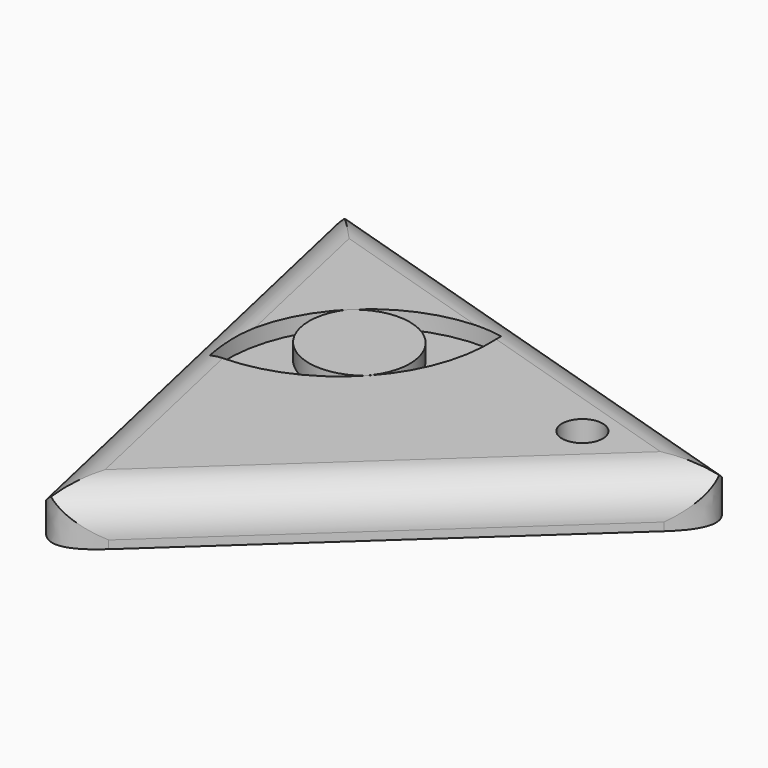
from build123d import *

# Parameters (mm, degrees)
F1_DEPTH    = 6
F3_DEPTH    = 2
F5_DEPTH    = 2
F6_T1_DEPTH = 95.6484477973
F6_T3_DEPTH = 95.6484477973
F6_T5_DEPTH = 95.6484477973
F7_T1_DEPTH = 44.3012701892
F8_R        = 2.5
F9_DEPTH    = 32.8


# Not quite as in the source:
# - a fillet or chamfer that OpenCascade refuses, or shapes differently, is made with other operations: its cross-section is extruded or revolved along the edge and cut away or added
# - a feature of the source that left no trace in its solid (it failed there, or was rolled back) is left out


with BuildPart() as f1:
    # F0 (on Top) → F1 (new body)
    with BuildSketch(Plane.XY):
        Polygon((-12.152816169, -38.9364026487), (39.7963219102, 8.9435537945), (-27.6435057413, 29.9928488542), align=None)
    extrude(amount=F1_DEPTH)

    # F2 (on face) → F3 (cut)
    with BuildSketch(Plane.XY.offset(6)):
        with BuildLine():
            ThreePointArc((-16.4638161659, -4.259868525), (-1.9528341067, 1.3079860402), (3.1085531227, 16.0032901913))
            ThreePointArc((3.1085531227, 16.0032901913), (-11.8846429173, 10.9012104958), (-16.4638161659, -4.259868525))
        make_face()
    extrude(amount=-F3_DEPTH, mode=Mode.SUBTRACT)

    # F6: fillet of radius 5 on 3 edges, made by hand

    # F6_s2 → F6_t1 (cut)
    with BuildSketch(Plane(origin=(-10.4861497959, 46.660444211, 0), x_dir=(0, 0, 1), z_dir=(0.2192644008, -0.9756654768, 0))):
        with BuildLine():
            ThreePointArc((1, 20.3944501768), (4.5355339059, 18.9299840827), (6, 15.3944501768))
            Line((6, 15.3944501768), (6, 20.3944501768))
            Line((6, 20.3944501768), (1, 20.3944501768))
        make_face()
    extrude(amount=F6_T1_DEPTH, mode=Mode.SUBTRACT)

    # F6_s4 → F6_t3 (cut)
    with BuildSketch(Plane(origin=(45.6522049365, -14.2489499944, 0), x_dir=(0, 0, 1), z_dir=(-0.9545832889, 0.2979441972, 0))):
        with BuildLine():
            ThreePointArc((1, 20.3944501768), (4.5355339059, 18.9299840827), (6, 15.3944501768))
            Line((6, 15.3944501768), (6, 20.3944501768))
            Line((6, 20.3944501768), (1, 20.3944501768))
        make_face()
    extrude(amount=F6_T3_DEPTH, mode=Mode.SUBTRACT)

    # F6_s6 → F6_t5 (cut)
    with BuildSketch(Plane(origin=(-35.1660551406, -32.4114942166, 0), x_dir=(0, 0, 1), z_dir=(0.7353188881, 0.6777212796, 0))):
        with BuildLine():
            ThreePointArc((1, 20.3944501768), (4.5355339059, 18.9299840827), (6, 15.3944501768))
            Line((6, 15.3944501768), (6, 20.3944501768))
            Line((6, 20.3944501768), (1, 20.3944501768))
        make_face()
    extrude(amount=F6_T5_DEPTH, mode=Mode.SUBTRACT)

    # F7: fillet of radius 5 on 3 edges, made by hand

    # F7_s2 → F7_t1 (cut)
    with BuildSketch(Plane.XY.offset(-21.6506350946)):
        with BuildLine():
            add(Edge.make_bspline(
                [(-25.7446203291, 21.5433379695), (-27.6435057413, 29.9928488542), (-19.3765719594, 27.4125764177)],
                knots=[0, 0, 0, 1, 1, 1], degree=2, weights=[1, 1, 1]))
            Line((-19.3765719594, 27.4125764177), (-27.6435057413, 29.9928488542))
            Line((-27.6435057413, 29.9928488542), (-25.7446203291, 21.5433379695))
        make_face()
        with BuildLine():
            add(Edge.make_bspline(
                [(-14.0517015812, -30.4868917639), (-12.152816169, -38.9364026487), (-5.7847677993, -33.0671642005)],
                knots=[0, 0, 0, 1, 1, 1], degree=2, weights=[1, 1, 1]))
            Line((-5.7847677993, -33.0671642005), (-12.152816169, -38.9364026487))
            Line((-12.152816169, -38.9364026487), (-14.0517015812, -30.4868917639))
        make_face()
        with BuildLine():
            add(Edge.make_bspline(
                [(33.4282735406, 3.0743153463), (39.7963219102, 8.9435537945), (31.5293881284, 11.523826231)],
                knots=[0, 0, 0, 1, 1, 1], degree=2, weights=[1, 1, 1]))
            Line((31.5293881284, 11.523826231), (39.7963219102, 8.9435537945))
            Line((39.7963219102, 8.9435537945), (33.4282735406, 3.0743153463))
        make_face()
    extrude(amount=F7_T1_DEPTH, mode=Mode.SUBTRACT)

    # F8 (on face) → F9 (cut)
    with BuildSketch(Plane.XY.offset(6)):
        with Locations((21.5296056122, 5.4111843929)):
            Circle(F8_R)
    extrude(amount=-F9_DEPTH, mode=Mode.SUBTRACT)


with BuildPart() as f5:
    # F4 (on face) → F5 (new body)
    with BuildSketch(Plane.XY.offset(4)):
        with BuildLine():
            ThreePointArc((-11.8846429173, 10.9012104958), (-11.0325286439, 1.8456155594), (-1.9528341067, 1.3079860402))
            ThreePointArc((-1.9528341067, 1.3079860402), (-2.2132820516, 10.9761296439), (-11.8846429173, 10.9012104958))
        make_face()
    extrude(amount=F5_DEPTH)


solid = Compound([f1.part, f5.part])
